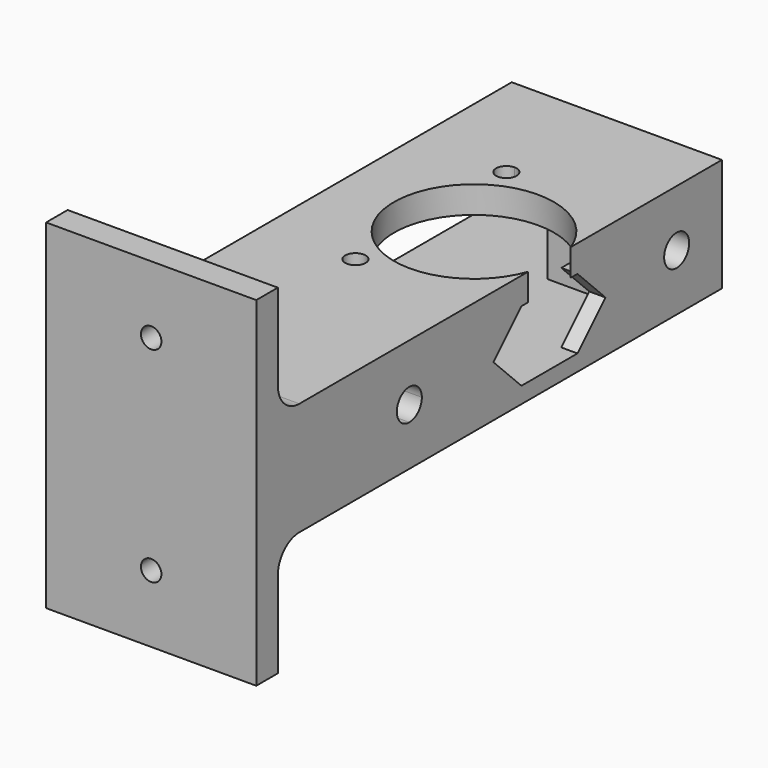
from build123d import *

# Parameters (mm, degrees)
F1_DEPTH  = 9
F2_W      = 39
F2_H      = 83
F3_DEPTH  = 5
F6_DEPTH  = 18
F7_W      = 18
F7_H      = 18
F8_DEPTH  = 18
F10_DEPTH = 3
F12_DEPTH = 5
F13_R     = 2.9
F14_DEPTH = 15
F15_W     = 3
F15_H     = 13
F16_DEPTH = 21
F17_DEPTH = 5
F18_W     = 39
F18_H     = 21
F19_DEPTH = 20
F21_DEPTH = 3
F22_R     = 5
F24_DEPTH = 25
F26_R     = 3.6982006044
F26_R_2   = 2.7022216625
F26_R_3   = 3.2521132856
F26_R_4   = 2.4365005618
F27_DEPTH = 3
F29_DEPTH = 25
F30_DEPTH = 2


# Not quite as in the source:
# - a pattern or mirror of a feature is missing from the dataset's text; its kind, count and spacing are read off the source's solid


with BuildPart() as f1:
    # F0 (on Top) → F1 (new body, symmetric)
    with BuildSketch(Plane.XY):
        Polygon((0, 0), (0, 83), (-3, 83), (-3, 3), (-39, 3), (-39, 0), align=None)
    extrude(amount=F1_DEPTH, both=True)

    # F2 (on face) → F3 (join)
    with BuildSketch(Plane.XY.offset(9)):
        with Locations((-19.5, 41.5)):
            Rectangle(F2_W, F2_H)
    extrude(amount=-F3_DEPTH)

    # F5 (on face) → F6 (join)
    with BuildSketch(Plane(origin=(0, 83, 0), x_dir=(-1, 0, 0), z_dir=(0, 1, 0))):
        Polygon((18, 9), (0, 9), (0, -9), (3, -9), (3, 4), (18, 4), align=None)
    extrude(amount=-F6_DEPTH)

    # F7 (on face) → F8 (join)
    with BuildSketch(Plane(origin=(0, 0, -9), x_dir=(1, 0, 0), z_dir=(0, 0, -1))):
        with Locations((-9, -9)):
            Rectangle(F7_W, F7_H)
    f8 = extrude(amount=-F8_DEPTH)

    # F8_copies: F8 across plane
    add(f8.mirror(Plane.ZX.offset(41.5)))

    # F9 (on face) → F10 (join)
    with BuildSketch(Plane(origin=(0, 0, -9), x_dir=(1, 0, 0), z_dir=(0, 0, -1))):
        Polygon((-22, -83), (0, -83), (0, 0), (-39, 0), (-39, -83), align=None)
    extrude(amount=F10_DEPTH)

    # F11 (on face) → F12 (cut, through all)
    with BuildSketch(Plane.XY.offset(9)):
        with BuildLine():
            Line((0, 38.0723795157), (0, 47.9276204843))
            ThreePointArc((0, 47.9276204843), (-28.8418814049, 43), (0, 38.0723795157))
        make_face()
    extrude(amount=-F12_DEPTH, mode=Mode.SUBTRACT)

    # F13 (on face) → F14 (cut)
    with BuildSketch(Plane.YZ):
        with BuildLine():
            Line((10.5, -1.5), (7.6, -1.5))
            ThreePointArc((7.6, -1.5), (8.4493903346, -3.5506096654), (10.5, -4.4))
            Line((10.5, -4.4), (10.5, -1.5))
        make_face()
        with BuildLine():
            ThreePointArc((13.4, -1.5), (10.5, 1.4), (7.6, -1.5))
            Line((7.6, -1.5), (10.5, -1.5))
            Line((10.5, -1.5), (10.5, -4.4))
            ThreePointArc((10.5, -4.4), (12.5506096654, -3.5506096654), (13.4, -1.5))
        make_face()
        Polygon((30, -2.5), (36.5, -9), (36.5, 4), align=None)
        Polygon((36.5, 4), (36.5, -9), (49.5, -9), (49.5, 4), (47.9276204843, 4), (38.0723795157, 4), align=None)
        Polygon((49.5, 4), (49.5, -9), (56, -2.5), align=None)
        with Locations((72.5, -1.5)):
            Circle(F13_R)
    extrude(amount=-F14_DEPTH, mode=Mode.SUBTRACT)

    # F15 (on face) → F16 (join, through all)
    with BuildSketch(Plane(origin=(-18, 0, 0), x_dir=(0, -1, 0), z_dir=(-1, 0, 0))):
        with Locations((-81.5, -2.5)):
            Rectangle(F15_W, F15_H)
    extrude(amount=F16_DEPTH)

    # F4 (on face) → F17 (cut, through all)
    with BuildSketch(Plane.XY.offset(9)):
        with BuildLine():
            ThreePointArc((-22, 62.4), (-23.3435028843, 59.1564971157), (-20.1, 60.5))
            ThreePointArc((-20.1, 60.5), (-20.6564971157, 61.8435028843), (-22, 62.4))
        make_face()
        with BuildLine():
            ThreePointArc((-22, 23.6), (-20.6564971157, 24.1564971157), (-20.1, 25.5))
            ThreePointArc((-20.1, 25.5), (-23.3435028843, 26.8435028843), (-22, 23.6))
        make_face()
    extrude(amount=-F17_DEPTH, mode=Mode.SUBTRACT)

    # F18 (on face) → F19 (join)
    with BuildSketch(Plane.XZ):
        with Locations((-19.5, -1.5)):
            Rectangle(F18_W, F18_H)
    extrude(amount=F19_DEPTH)

    # F20 (on face) → F21 (join)
    with BuildSketch(Plane.XZ.offset(20)):
        Polygon((0, 30), (-39, 30), (-39, 9), (-39, -12), (-39, -33), (0, -33), (0, -12), (0, 9), align=None)
    extrude(amount=F21_DEPTH)

    # F22
    f22_edges = [f1.edges().sort_by_distance(p)[0] for p in [
        (-19.5, -20, -12),
        (-19.5, -20, 9),
    ]]
    fillet(f22_edges, radius=F22_R)

    # F23 (on face) → F24 (cut)
    with BuildSketch(Plane.XZ.offset(23)):
        with BuildLine():
            Line((-32, 21.1), (-32, 23))
            Line((-32, 23), (-30.1, 23))
            ThreePointArc((-30.1, 23), (-33.3435028843, 24.3435028843), (-32, 21.1))
        make_face()
        with BuildLine():
            Line((-30.1, 23), (-32, 23))
            Line((-32, 23), (-32, 21.1))
            ThreePointArc((-32, 21.1), (-30.6564971157, 21.6564971157), (-30.1, 23))
        make_face()
        with BuildLine():
            ThreePointArc((-5.1, 23), (-7, 24.9), (-8.9, 23))
            Line((-8.9, 23), (-7, 23))
            Line((-7, 23), (-7, 21.1))
            ThreePointArc((-7, 21.1), (-5.6564971157, 21.6564971157), (-5.1, 23))
        make_face()
        with BuildLine():
            Line((-7, 23), (-8.9, 23))
            ThreePointArc((-8.9, 23), (-8.3435028843, 21.6564971157), (-7, 21.1))
            Line((-7, 21.1), (-7, 23))
        make_face()
        with BuildLine():
            Line((-32, -26), (-32, -24.1))
            ThreePointArc((-32, -24.1), (-33.3435028843, -27.3435028843), (-30.1, -26))
            Line((-30.1, -26), (-32, -26))
        make_face()
        with BuildLine():
            ThreePointArc((-30.1, -26), (-30.6564971157, -24.6564971157), (-32, -24.1))
            Line((-32, -24.1), (-32, -26))
            Line((-32, -26), (-30.1, -26))
        make_face()
        with BuildLine():
            ThreePointArc((-5.1, -26), (-5.6564971157, -24.6564971157), (-7, -24.1))
            Line((-7, -24.1), (-7, -26))
            Line((-7, -26), (-8.9, -26))
            ThreePointArc((-8.9, -26), (-7, -27.9), (-5.1, -26))
        make_face()
        with BuildLine():
            Line((-7, -26), (-7, -24.1))
            ThreePointArc((-7, -24.1), (-8.3435028843, -24.6564971157), (-8.9, -26))
            Line((-8.9, -26), (-7, -26))
        make_face()
    extrude(amount=-F24_DEPTH, mode=Mode.SUBTRACT)

    # F26 (on face) → F27 (join, through all)
    with BuildSketch(Plane(origin=(0, -20, 0), x_dir=(-1, 0, 0), z_dir=(0, 1, 0))):
        with Locations((32, 23)):
            Circle(F26_R)
        with Locations((7, 23)):
            Circle(F26_R_2)
        with Locations((31.5193422139, -25.7969032973)):
            Circle(F26_R_3)
        with Locations((7.0765195414, -26.2656044215)):
            Circle(F26_R_4)
    extrude(amount=-F27_DEPTH)

    # F28 (on face) → F29 (cut)
    with BuildSketch(Plane(origin=(0, -20, 0), x_dir=(-1, 0, 0), z_dir=(0, 1, 0))):
        with BuildLine():
            ThreePointArc((19.5, 15.6), (20.8435028843, 16.1564971157), (21.4, 17.5))
            ThreePointArc((21.4, 17.5), (20.8435028843, 18.8435028843), (19.5, 19.4))
            Line((19.5, 19.4), (19.5, 17.5))
            Line((19.5, 17.5), (19.5, 15.6))
        make_face()
        with BuildLine():
            ThreePointArc((21.4, -20.5), (20.8435028843, -19.1564971157), (19.5, -18.6))
            Line((19.5, -18.6), (19.5, -20.5))
            Line((19.5, -20.5), (19.5, -22.4))
            ThreePointArc((19.5, -22.4), (20.8435028843, -21.8435028843), (21.4, -20.5))
        make_face()
        with BuildLine():
            Line((19.5, -20.5), (19.5, -18.6))
            ThreePointArc((19.5, -18.6), (17.6, -20.5), (19.5, -22.4))
            Line((19.5, -22.4), (19.5, -20.5))
        make_face()
        with BuildLine():
            Line((19.5, 17.5), (19.5, 19.4))
            ThreePointArc((19.5, 19.4), (17.6, 17.5), (19.5, 15.6))
            Line((19.5, 15.6), (19.5, 17.5))
        make_face()
    extrude(amount=-F29_DEPTH, mode=Mode.SUBTRACT)

    # F30 (add): a face of the model
    f30_faces = [f1.faces().sort_by_distance(p)[0] for p in [
        (-19.5, -23, -1.5),
    ]]
    extrude(f30_faces, amount=F30_DEPTH)


solid = f1.part
